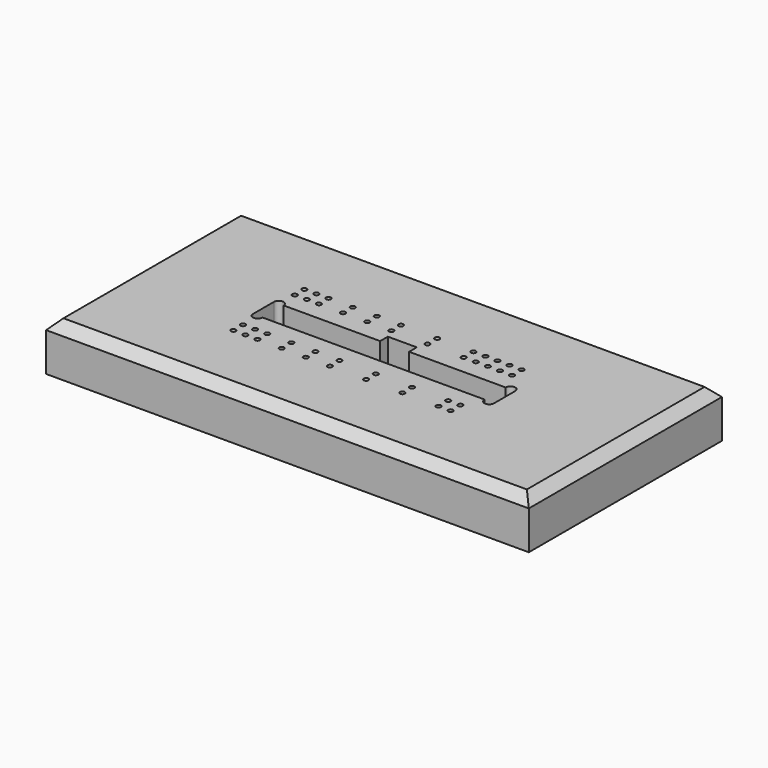
from build123d import *

# Parameters (mm, degrees)
F0_W     = 100
F0_H     = 50
F1_DEPTH = 10
F3_DEPTH = 5
F4_R     = 0.5
F5_DEPTH = 10.001
F6_SIZE  = 2


# Not quite as in the source:
# - a feature names something its author has since deleted; it is built from what else it names


with BuildPart() as f1:
    # F0 (on Top) → F1 (new body)
    with BuildSketch(Plane.XY):
        with Locations((50, 25)):
            Rectangle(F0_W, F0_H)
    extrude(amount=F1_DEPTH)

    # F2 (on face) → F3 (cut)
    with BuildSketch(Plane.XY.offset(10)):
        with BuildLine():
            ThreePointArc((25, 22.3178226352), (26, 21.3178226352), (27, 22.3178226352))
            Line((27, 22.3178226352), (73.0023026059, 22.3178226352))
            ThreePointArc((73.0023026059, 22.3178226352), (73.9660691444, 21.2505758173), (75, 22.25))
            Line((75, 22.25), (75, 27.75))
            ThreePointArc((75, 27.75), (74, 28.75), (73, 27.75))
            Line((73, 27.75), (53, 27.75))
            Line((53, 27.75), (53, 29.75))
            Line((53, 29.75), (47, 29.75))
            Line((47, 29.75), (47, 27.75))
            Line((47, 27.75), (27, 27.75))
            ThreePointArc((27, 27.75), (26, 28.75), (25, 27.75))
            Line((25, 27.75), (25, 22.3178226352))
        make_face()
    extrude(amount=-F3_DEPTH, mode=Mode.SUBTRACT)

    # F4 (on face) → F5 (cut, through all)
    with BuildSketch(Plane.XY.offset(10)):
        with Locations((26.13, 31.7288823426)):
            Circle(F4_R)
        with Locations((28.63, 31.7288823426)):
            Circle(F4_R)
        with Locations((31.13, 31.7288823426)):
            Circle(F4_R)
        with Locations((36.13, 31.7288823426)):
            Circle(F4_R)
        with Locations((41.13, 31.7288823426)):
            Circle(F4_R)
        with Locations((46.13, 31.7288823426)):
            Circle(F4_R)
        with Locations((53.63, 31.7288823426)):
            Circle(F4_R)
        with Locations((61.13, 31.7288823426)):
            Circle(F4_R)
        with Locations((63.63, 31.7288823426)):
            Circle(F4_R)
        with Locations((66.13, 31.7288823426)):
            Circle(F4_R)
        with Locations((68.63, 31.7288823426)):
            Circle(F4_R)
        with Locations((71.13, 31.7288823426)):
            Circle(F4_R)
        with Locations((71.13, 18.3389402926)):
            Circle(F4_R)
        with Locations((61.13, 18.3389402926)):
            Circle(F4_R)
        with Locations((26.13, 18.3389402926)):
            Circle(F4_R)
        with Locations((28.63, 18.3389402926)):
            Circle(F4_R)
        with Locations((31.13, 18.3389402926)):
            Circle(F4_R)
        with Locations((36.13, 18.3389402926)):
            Circle(F4_R)
        with Locations((41.13, 18.3389402926)):
            Circle(F4_R)
        with Locations((46.13, 18.3389402926)):
            Circle(F4_R)
        with Locations((53.63, 18.3389402926)):
            Circle(F4_R)
        with Locations((68.63, 18.3389402926)):
            Circle(F4_R)
        with Locations((26.13, 34.2288823426)):
            Circle(F4_R)
        with Locations((28.63, 34.2288823426)):
            Circle(F4_R)
        with Locations((31.13, 34.2288823426)):
            Circle(F4_R)
        with Locations((36.13, 34.2288823426)):
            Circle(F4_R)
        with Locations((41.13, 34.2288823426)):
            Circle(F4_R)
        with Locations((46.13, 34.2288823426)):
            Circle(F4_R)
        with Locations((53.63, 34.2288823426)):
            Circle(F4_R)
        with Locations((61.13, 34.2288823426)):
            Circle(F4_R)
        with Locations((63.63, 34.2288823426)):
            Circle(F4_R)
        with Locations((66.13, 34.2288823426)):
            Circle(F4_R)
        with Locations((68.63, 34.2288823426)):
            Circle(F4_R)
        with Locations((71.13, 34.2288823426)):
            Circle(F4_R)
        with Locations((41.13, 15.8389402926)):
            Circle(F4_R)
        with Locations((61.13, 15.8389402926)):
            Circle(F4_R)
        with Locations((36.13, 15.8389402926)):
            Circle(F4_R)
        with Locations((53.63, 15.8389402926)):
            Circle(F4_R)
        with Locations((46.13, 15.8389402926)):
            Circle(F4_R)
        with Locations((71.13, 15.8389402926)):
            Circle(F4_R)
        with Locations((31.13, 15.8389402926)):
            Circle(F4_R)
        with Locations((26.13, 15.8389402926)):
            Circle(F4_R)
        with Locations((68.63, 15.8389402926)):
            Circle(F4_R)
        with Locations((28.63, 15.8389402926)):
            Circle(F4_R)
    extrude(amount=-F5_DEPTH, mode=Mode.SUBTRACT)

    # F6
    f6_edges = [f1.edges().sort_by_distance(p)[0] for p in [
        (50, 0, 10),
        (0, 25, 10),
        (50, 50, 10),
        (100, 25, 10),
    ]]
    chamfer(f6_edges, length=F6_SIZE)


solid = f1.part
